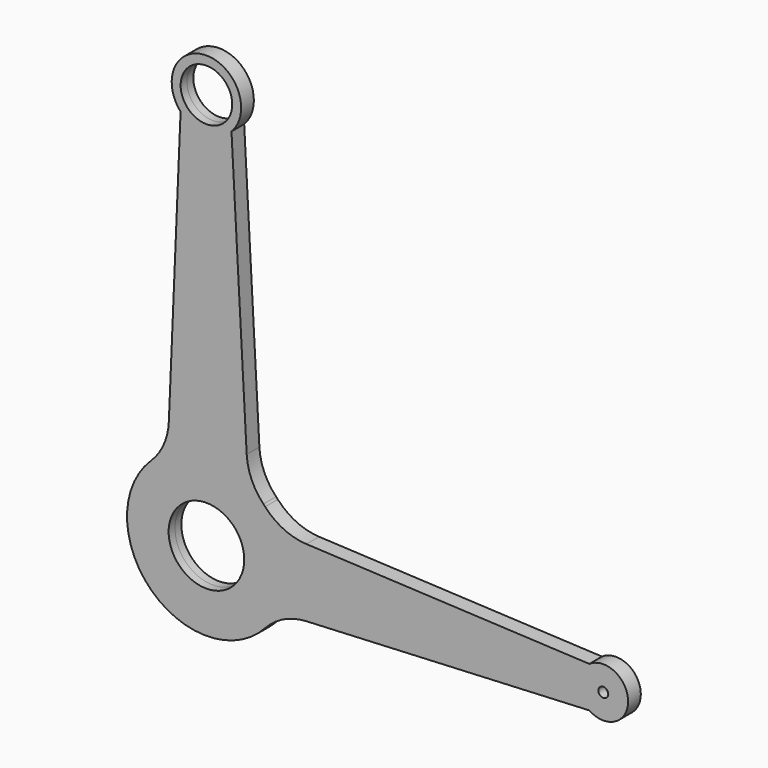
from build123d import *

# Parameters (mm, degrees)
F0_R        = 19.0457812865
F0_R_2      = 13
F0_R_3      = 2.5
F1_DEPTH    = 4
F2_R        = 30
F3_R        = 30
F4_T1_DEPTH = 8
F5_R        = 30


# Not quite as in the source:
# - a fillet or chamfer that OpenCascade refuses, or shapes differently, is made with other operations: its cross-section is extruded or revolved along the edge and cut away or added


with BuildPart() as f1:
    # F0 (on Front) → F1 (new body, symmetric)
    with BuildSketch(Plane.XZ):
        with BuildLine():
            ThreePointArc((-19.5365896508, 34.9044648264), (0.8487956626, 39.99099331), (21, 34.0440890611))
            Line((21, 34.0440890611), (12.6265428967, 187.8830525924))
            ThreePointArc((12.6265428967, 187.8830525924), (-0.2904480488, 182.5024104537), (-13.0217419566, 188.3087966224))
            Line((-13.0217419566, 188.3087966224), (-19.5365896508, 34.9044648264))
        make_face()
        with BuildLine():
            ThreePointArc((35.8133699363, 17.8157945038), (38.939278354, 9.1505519655), (40, 0))
            ThreePointArc((40, 0), (38.9395050251, -9.1495873352), (35.8142525798, -17.8140201007))
            Line((35.8142525798, -17.8140201007), (192.9463185859, -10.3196694961))
            ThreePointArc((192.9463185859, -10.3196694961), (187.5000024995, 0.0079048318), (192.9593762653, 10.3285825468))
            Line((192.9593762653, 10.3285825468), (35.8133699363, 17.8157945038))
        make_face()
        with BuildLine():
            ThreePointArc((35.8142525798, -17.8140201007), (38.9395050251, -9.1495873352), (40, 0))
            ThreePointArc((40, 0), (38.939278354, 9.1505519655), (35.8133699363, 17.8157945038))
            ThreePointArc((35.8133699363, 17.8157945038), (29.542835628, 26.9670328931), (21, 34.0440890611))
            ThreePointArc((21, 34.0440890611), (0.8487956626, 39.99099331), (-19.5365896508, 34.9044648264))
            ThreePointArc((-19.5365896508, 34.9044648264), (-27.5871390481, -28.9646294494), (35.8142525798, -17.8140201007))
        make_face()
        Circle(F0_R, mode=Mode.SUBTRACT)
        with BuildLine():
            ThreePointArc((-13.0217419566, 188.3087966224), (-0.2904480488, 182.5024104537), (12.6265428967, 187.8830525924))
            ThreePointArc((12.6265428967, 187.8830525924), (16.2359862757, 193.4698583741), (17.5, 200))
            ThreePointArc((17.5, 200), (-6.2597729895, 216.3421308929), (-13.0217419566, 188.3087966224))
        make_face()
        with Locations((0, 200)):
            Circle(F0_R_2, mode=Mode.SUBTRACT)
        with BuildLine():
            ThreePointArc((212.5, 0), (205.841327046, 11.0511944306), (192.9593762653, 10.3285825468))
            ThreePointArc((192.9593762653, 10.3285825468), (187.5000024995, 0.0079048318), (192.9463185859, -10.3196694961))
            ThreePointArc((192.9463185859, -10.3196694961), (205.8343372513, -11.0548861974), (212.5, 0))
        make_face()
        with Locations((200, 0)):
            Circle(F0_R_3, mode=Mode.SUBTRACT)
    extrude(amount=F1_DEPTH, both=True)

    # F2
    f2_edges = [f1.edges().sort_by_distance(p)[0] for p in [
        (35.81337, 0, 17.815795),
    ]]
    fillet(f2_edges, radius=F2_R)

    # F3
    f3_edges = [f1.edges().sort_by_distance(p)[0] for p in [
        (21, 0, 34.044089),
    ]]
    fillet(f3_edges, radius=F3_R)

    # F4: fillet of radius 30 on 1 edges, made by hand

    # F4_s2 → F4_t1 (join)
    with BuildSketch(Plane.XZ.offset(-4)):
        with BuildLine():
            ThreePointArc((-18.9466482885, 48.7957428331), (-21.5235892515, 37.8433937284), (-27.954075006, 28.6106569403))
            ThreePointArc((-27.954075006, 28.6106569403), (-23.9529499606, 32.0352335435), (-19.5365896508, 34.9044648264))
            Line((-19.5365896508, 34.9044648264), (-18.9466482885, 48.7957428331))
        make_face()
    extrude(amount=F4_T1_DEPTH)

    # F5
    f5_edges = [f1.edges().sort_by_distance(p)[0] for p in [
        (35.814253, 0, -17.81402),
    ]]
    fillet(f5_edges, radius=F5_R)


solid = f1.part
